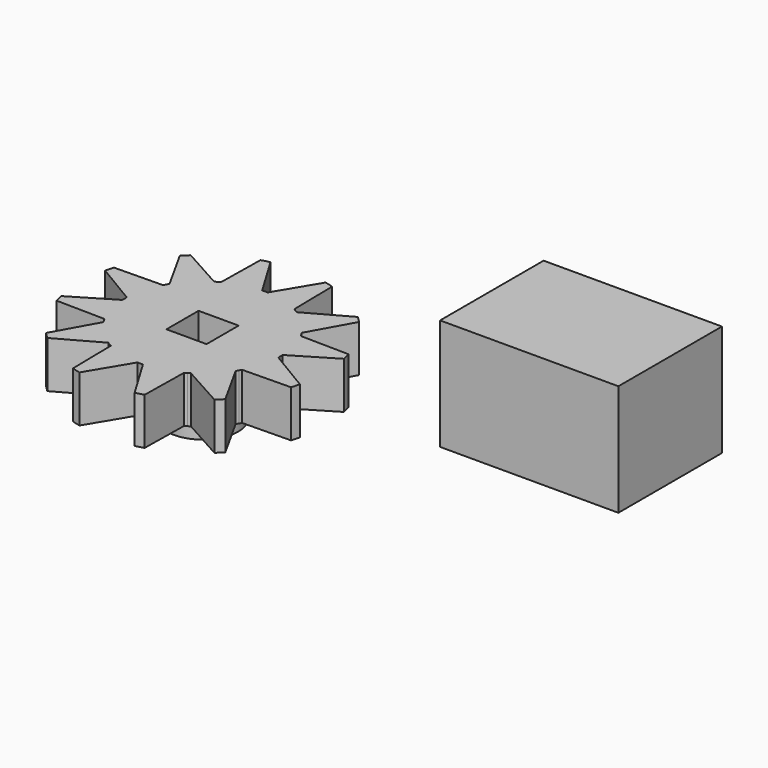
from build123d import *

# Parameters (mm, degrees)
F0_R            = 11
F1_DEPTH        = 4.2
F3_DEPTH        = 4.201
F3_COPIES_COUNT = 12
F5_R            = 3.2
F6_DEPTH        = 3
F7_W            = 3.6
F7_H            = 3.6
F8_DEPTH        = 7.201
F9_W            = 16.0063430667
F9_H            = 11.617815122
F10_DEPTH       = 10


# Not quite as in the source:
# - a pattern or mirror of a feature is missing from the dataset's text; its kind, count and spacing are read off the source's solid


with BuildPart() as f1:
    # F0 (on Top) → F1 (new body)
    with BuildSketch(Plane.XY):
        Circle(F0_R)
    extrude(amount=F1_DEPTH)

    # F2 (on face) → F3 (cut, through all)
    with BuildSketch(Plane.XY.offset(4.2)):
        with BuildLine():
            ThreePointArc((0.2442964769, -6.9957357891), (0.1221668451, -6.9989338661), (0, -7))
            Line((0, -7), (0, -11))
            ThreePointArc((0, -11), (1.2452353514, -10.9292904124), (2.4744615978, -10.7180707126))
            Line((2.4744615978, -10.7180707126), (0.2442964769, -6.9957357891))
        make_face()
        with BuildLine():
            Line((0, -11), (0, -7))
            ThreePointArc((0, -7), (-0.1221668451, -6.9989338661), (-0.2442964769, -6.9957357891))
            Line((-0.2442964769, -6.9957357891), (-2.4744615978, -10.7180707126))
            ThreePointArc((-2.4744615978, -10.7180707126), (-1.2452353514, -10.9292904124), (0, -11))
        make_face()
    f3 = extrude(amount=-F3_DEPTH, mode=Mode.SUBTRACT)

    # F3_copies: F3 ×12 about axis
    f3_copies_axis = Axis((0, 0, 0), (0, 0, 1))
    for i in range(1, F3_COPIES_COUNT):
        add(f3.rotate(f3_copies_axis, i * 360 / F3_COPIES_COUNT), mode=Mode.SUBTRACT)

    # F5 (on face) → F6 (join)
    with BuildSketch(Plane(origin=(0, 0, 0), x_dir=(1, 0, 0), z_dir=(0, 0, -1))):
        Circle(F5_R)
    extrude(amount=F6_DEPTH)

    # F7 (on face) → F8 (cut, through all)
    with BuildSketch(Plane(origin=(0, 0, -3), x_dir=(1, 0, 0), z_dir=(0, 0, -1))):
        Rectangle(F7_W, F7_H)
    extrude(amount=-F8_DEPTH, mode=Mode.SUBTRACT)


with BuildPart() as f10:
    # F9 (on Top) → F10 (new body)
    with BuildSketch(Plane.XY):
        with Locations((27.296114713, 8.3463508636)):
            Rectangle(F9_W, F9_H)
    extrude(amount=F10_DEPTH)


solid = Compound([f1.part, f10.part])
